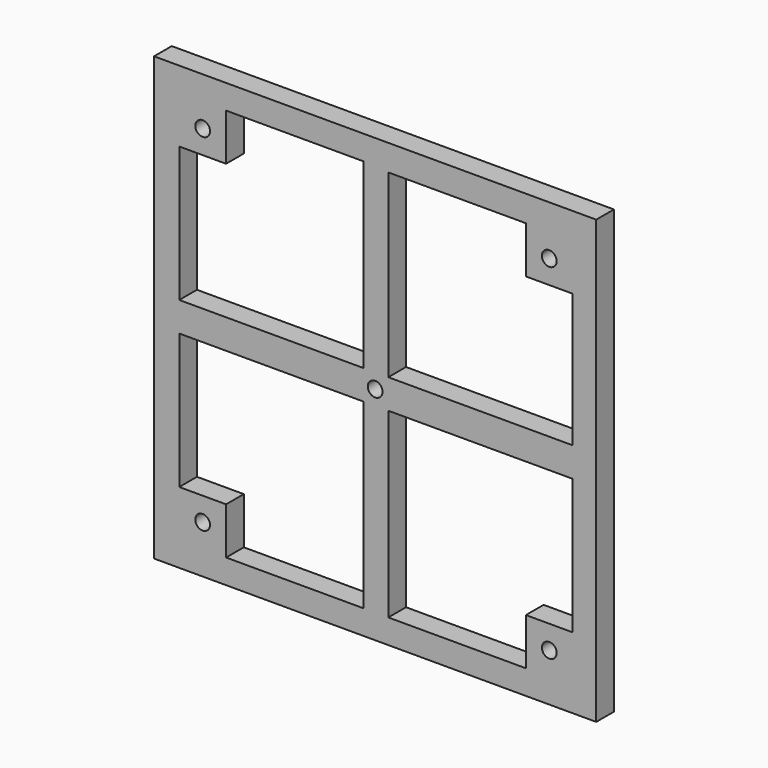
from build123d import *

# Parameters (mm, degrees)
F0_W     = 59.944
F0_H     = 59.944
F0_W_2   = 25
F0_H_2   = 2
F0_W_3   = 6.35
F0_H_3   = 6.35
F1_DEPTH = 3
F2_D     = 2


# Not quite as in the source:
# - a feature names something its author has since deleted; it is built from what else it names


with BuildPart() as f1:
    # F0 (on Front) → F1 (new body)
    with BuildSketch(Plane.XZ):
        Rectangle(F0_W, F0_H)
        Polygon((-26.5568002729, 26.67), (-20.2068002729, 26.67), (-1.5568002729, 26.67), (-1.5568002729, 20.32), (-1.5568002729, 2), (-1.5568002729, 0), (-1.5568002729, -2), (-1.5568002729, -20.32), (-1.5568002729, -26.67), (-20.2068002729, -26.67), (-26.5568002729, -26.67), (-26.5568002729, -20.32), (-26.5568002729, -2), (-26.5568002729, 0), (-26.5568002729, 2), (-26.5568002729, 20.32), align=None, mode=Mode.SUBTRACT)
        Polygon((20.4331997271, 26.4424991059), (26.7831997271, 26.4424991059), (26.7831997271, 20.0924991059), (26.7831997271, 2), (26.7831997271, 0), (26.7831997271, -2), (26.7831997271, -20.32), (26.7831997271, -26.67), (20.4331997271, -26.67), (1.7831997271, -26.67), (1.7831997271, -20.32), (1.7831997271, -2), (1.7831997271, 0), (1.7831997271, 2), (1.7831997271, 20.0924991059), (1.7831997271, 26.4424991059), align=None, mode=Mode.SUBTRACT)
        with Locations((14.2831997271, 1)):
            Rectangle(F0_W_2, F0_H_2)
        with Locations((14.2831997271, -1)):
            Rectangle(F0_W_2, F0_H_2)
        with Locations((-14.0568002729, 1)):
            Rectangle(F0_W_2, F0_H_2)
        with Locations((-14.0568002729, -1)):
            Rectangle(F0_W_2, F0_H_2)
        Polygon((-20.2068002729, 26.4424991059), (-20.2068002729, 26.67), (-26.5568002729, 26.67), (-26.5568002729, 20.32), (-20.2068002729, 20.32), align=None)
        Polygon((26.7831997271, 20.0924991059), (26.7831997271, 26.4424991059), (20.4331997271, 26.4424991059), (20.4331997271, 20.32), (20.4331997271, 20.0924991059), align=None)
        with Locations((23.6081997271, -23.495)):
            Rectangle(F0_W_3, F0_H_3)
        with Locations((-23.3818002729, -23.495)):
            Rectangle(F0_W_3, F0_H_3)
    extrude(amount=F1_DEPTH)

    # F2 (through all)
    with Locations(Plane(origin=(0, 0, 0), x_dir=(1, 0, 0), z_dir=(0, 1, 0))):
        with Locations((23.6081997271, -23.2674991059), (0, 0), (23.6081997271, 23.495), (-23.3818002729, -23.495), (-23.3818002729, 23.495)):
            Hole(F2_D / 2)


solid = f1.part
